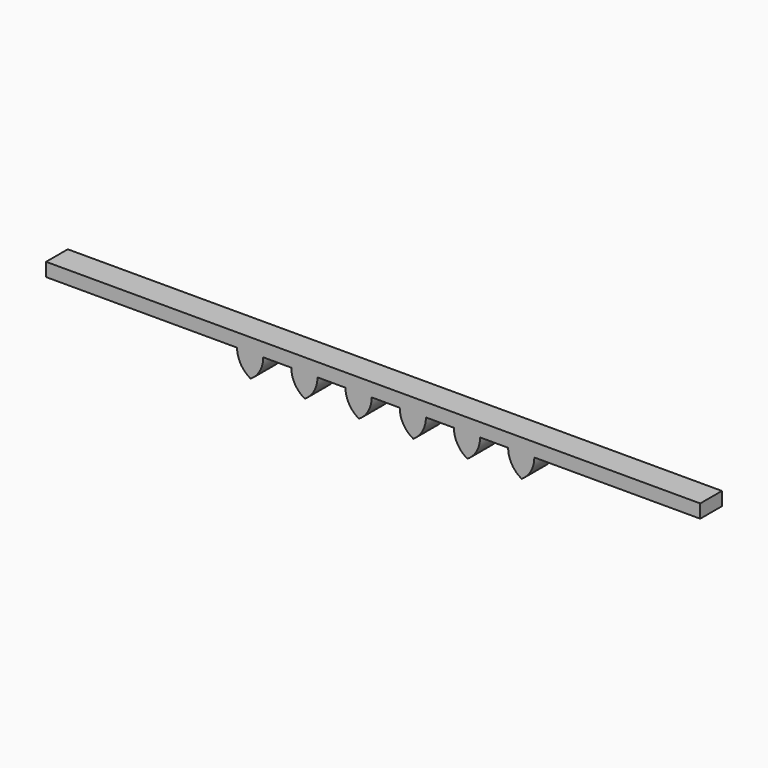
from build123d import *

# Parameters (mm, degrees)
F1_DEPTH = 6.35


# Not quite as in the source:
# - a feature names something its author has since deleted; it is built from what else it names


with BuildPart() as f1:
    # F0 (on Front) → F1 (new body)
    with BuildSketch(Plane.XZ):
        with BuildLine():
            Line((-82.3832392616, 36.3007842489), (-88.5181630436, 36.3007842489))
            ThreePointArc((-88.5181630436, 36.3007842489), (-87.6661618487, 33.1818070528), (-85.3468053884, 30.9291396569))
            ThreePointArc((-85.3468053884, 30.9291396569), (-83.1732772521, 33.2333223579), (-82.3832392616, 36.3007842489))
        make_face()
        with BuildLine():
            Line((-69.6832392616, 36.3007842489), (-75.8181630436, 36.3007842489))
            ThreePointArc((-75.8181630436, 36.3007842489), (-74.9661618487, 33.1818070528), (-72.6468053884, 30.9291396569))
            ThreePointArc((-72.6468053884, 30.9291396569), (-70.4732772521, 33.2333223579), (-69.6832392616, 36.3007842489))
        make_face()
        with BuildLine():
            Line((-56.9832392616, 36.3007842489), (-63.1181630436, 36.3007842489))
            ThreePointArc((-63.1181630436, 36.3007842489), (-62.2661618487, 33.1818070528), (-59.9468053884, 30.9291396569))
            ThreePointArc((-59.9468053884, 30.9291396569), (-57.7732772521, 33.2333223579), (-56.9832392616, 36.3007842489))
        make_face()
        with BuildLine():
            Line((-44.2832392616, 36.3007842489), (-50.4181630436, 36.3007842489))
            ThreePointArc((-50.4181630436, 36.3007842489), (-49.5661618487, 33.1818070528), (-47.2468053884, 30.9291396569))
            ThreePointArc((-47.2468053884, 30.9291396569), (-45.0732772521, 33.2333223579), (-44.2832392616, 36.3007842489))
        make_face()
        with BuildLine():
            Line((-31.5832392616, 36.3007842489), (-37.7181630436, 36.3007842489))
            ThreePointArc((-37.7181630436, 36.3007842489), (-36.8661618487, 33.1818070528), (-34.5468053884, 30.9291396569))
            ThreePointArc((-34.5468053884, 30.9291396569), (-32.3732772521, 33.2333223579), (-31.5832392616, 36.3007842489))
        make_face()
        with BuildLine():
            Line((-18.8832392616, 36.3007842489), (-25.0181630436, 36.3007842489))
            ThreePointArc((-25.0181630436, 36.3007842489), (-24.1661618487, 33.1818070528), (-21.8468053884, 30.9291396569))
            ThreePointArc((-21.8468053884, 30.9291396569), (-19.6732772521, 33.2333223579), (-18.8832392616, 36.3007842489))
        make_face()
        Polygon((-117.1290501952, 36.3007842489), (-100.1673217514, 36.3007842489), (-88.5181630436, 36.3007842489), (-82.3832392616, 36.3007842489), (-75.8181630436, 36.3007842489), (-69.6832392616, 36.3007842489), (-63.1181630436, 36.3007842489), (-56.9832392616, 36.3007842489), (-50.4181630436, 36.3007842489), (-44.2832392616, 36.3007842489), (-37.7181630436, 36.3007842489), (-31.5832392616, 36.3007842489), (-25.0181630436, 36.3007842489), (-18.8832392616, 36.3007842489), (1.4326782486, 36.3007842489), (15.6819988042, 36.3007842489), (19.9843030423, 36.3007842489), (19.9843030423, 39.4588721526), (6.4166695811, 39.4588721526), (1.4326782486, 39.4588721526), (-106.9938540459, 39.4588721526), (-120.9527105093, 39.4588721526), (-133.2595199347, 39.4588721526), (-133.2595199347, 36.3007842489), (-127.7280002832, 36.3007842489), align=None)
    extrude(amount=F1_DEPTH)


solid = f1.part
